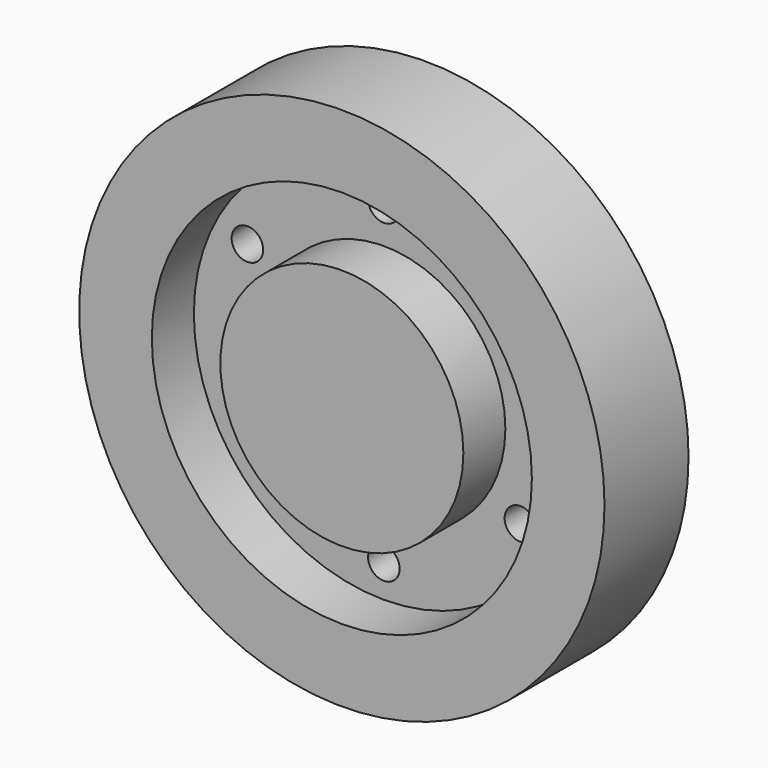
from build123d import *

# Parameters (mm, degrees)
F0_R            = 63.5
F1_DEPTH        = 25.4
F2_R            = 45.938884012
F2_R_2          = 29.3747144419
F3_DEPTH        = 12.7
F4_R            = 3.81
F5_DEPTH        = 12.701
F5_COPIES_COUNT = 6


# Not quite as in the source:
# - a pattern or mirror of a feature is missing from the dataset's text; its kind, count and spacing are read off the source's solid


with BuildPart() as f1:
    # F0 (on Front) → F1 (new body)
    with BuildSketch(Plane.XZ):
        Circle(F0_R)
    extrude(amount=F1_DEPTH)

    # F2 (on face) → F3 (cut)
    with BuildSketch(Plane.XZ.offset(25.4)):
        Circle(F2_R)
        Circle(F2_R_2, mode=Mode.SUBTRACT)
    extrude(amount=-F3_DEPTH, mode=Mode.SUBTRACT)

    # F4 (on face) → F5 (cut, through all)
    with BuildSketch(Plane.XZ.offset(12.7)):
        with Locations((0, 38.1)):
            Circle(F4_R)
    f5 = extrude(amount=-F5_DEPTH, mode=Mode.SUBTRACT)

    # F5_copies: F5 ×6 about axis
    f5_copies_axis = Axis((0, 0, 0), (0, 1, 0))
    for i in range(1, F5_COPIES_COUNT):
        add(f5.rotate(f5_copies_axis, i * 360 / F5_COPIES_COUNT), mode=Mode.SUBTRACT)


solid = f1.part
